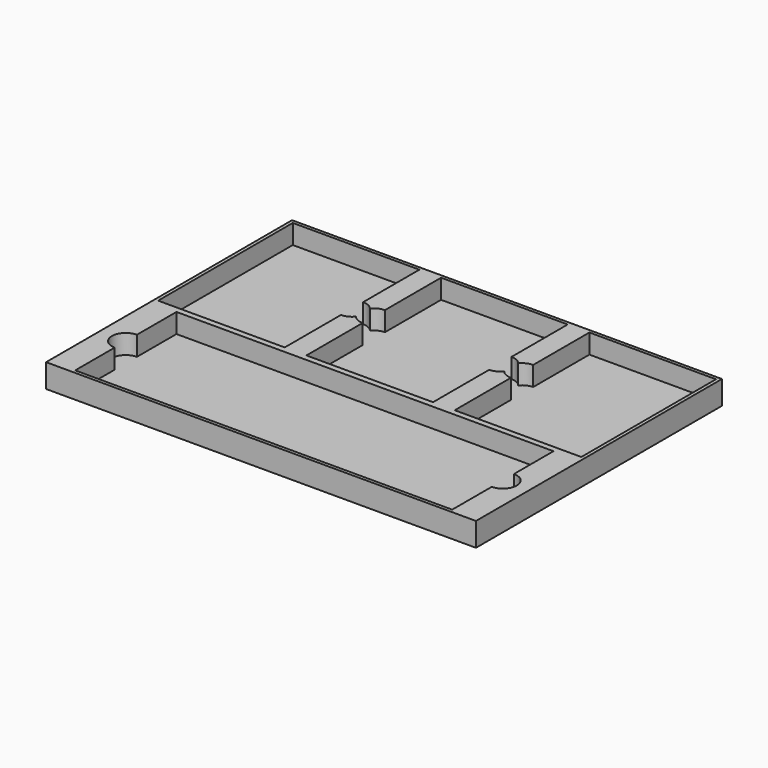
from build123d import *

# Parameters (mm, degrees)
F1_DEPTH = 3
F2_DEPTH = 17


# Not quite as in the source:
# - ends of sketch curves that miss each other by under 0.0002 mm in the source are joined


with BuildPart() as f1:
    # F0 (on Top) → F1 (new body)
    with BuildSketch(Plane.XY):
        Polygon((154.5, 110.5), (-154.5, 110.5), (-154.4999927282, -110.5), (154.5, -110.5), align=None)
        with BuildLine():
            Line((135.5, -108.0998892117), (-135.5, -108.0998892117))
            Line((-135.5, -108.0998892117), (-135.5, -72.5998892117))
            ThreePointArc((-135.5, -72.5998892117), (-145.5, -62.5998892117), (-135.5, -52.5998892117))
            Line((-135.5, -52.5998892117), (-135.5, -17.0998892117))
            Line((-135.5, -17.0998892117), (135.5, -17.0998892117))
            Line((135.5, -17.0998892117), (135.5, -52.5998892117))
            ThreePointArc((135.5, -52.5998892117), (142.5710678119, -55.5288213998), (145.5, -62.5998892117))
            ThreePointArc((145.5, -62.5998892117), (142.5710678119, -69.6709570235), (135.5, -72.5998892117))
            Line((135.5, -72.5998892117), (135.5, -108.0998892117))
        make_face(mode=Mode.SUBTRACT)
        with BuildLine():
            Line((-45.4999990761, 57.6660784096), (-45.4999990761, 108.1660784096))
            Line((-45.4999990761, 108.1660784096), (45.5000009239, 108.1660784096))
            Line((45.5000009239, 108.1660784096), (45.5000009239, 57.6660784096))
            ThreePointArc((45.5000009239, 57.6660784096), (49.8255857676, 56.6821371804), (53.2999463577, 53.9239415616))
            ThreePointArc((53.2999463577, 53.9239415616), (56.7743069478, 56.6821371804), (61.0998917915, 57.6660784096))
            Line((61.0998917915, 57.6660784096), (61.0998917915, 108.1660784096))
            Line((61.0998917915, 108.1660784096), (152.0998917915, 108.1660784096))
            Line((152.0998917915, 108.1660784096), (152.0998917915, -12.8339215904))
            Line((152.0998917915, -12.8339215904), (61.0998917915, -12.8339215904))
            Line((61.0998917915, -12.8339215904), (61.0998917915, 37.6660784096))
            ThreePointArc((61.0998917915, 37.6660784096), (56.7743069478, 38.6500196387), (53.2999463577, 41.4082152575))
            ThreePointArc((53.2999463577, 41.4082152575), (49.8255857676, 38.6500196387), (45.5000009239, 37.6660784096))
            Line((45.5000009239, 37.6660784096), (45.5000009239, -12.8339215904))
            Line((45.5000009239, -12.8339215904), (-45.4999990761, -12.8339215904))
            Line((-45.4999990761, -12.8339215904), (-45.4999990761, 37.6660784096))
            ThreePointArc((-45.4999990761, 37.6660784096), (-49.8257290565, 38.6500892715), (-53.3001459795, 41.4084663822))
            ThreePointArc((-53.3001459795, 41.4084663822), (-56.7745629026, 38.6500892715), (-61.1002928829, 37.6660784096))
            Line((-61.1002928829, 37.6660784096), (-61.1002928829, -12.8339215904))
            Line((-61.1002928829, -12.8339215904), (-152.1002928829, -12.8339215904))
            Line((-152.1002928829, -12.8339215904), (-152.1002928829, 108.1660784096))
            Line((-152.1002928829, 108.1660784096), (-61.1002928829, 108.1660784096))
            Line((-61.1002928829, 108.1660784096), (-61.1002928829, 57.6660784096))
            ThreePointArc((-61.1002928829, 57.6660784096), (-56.7745629026, 56.6820675476), (-53.3001459795, 53.923690437))
            ThreePointArc((-53.3001459795, 53.923690437), (-49.8257290565, 56.6820675476), (-45.4999990761, 57.6660784096))
        make_face(mode=Mode.SUBTRACT)
        with BuildLine():
            Line((-135.5, -72.5998892117), (-135.5, -108.0998892117))
            Line((-135.5, -108.0998892117), (135.5, -108.0998892117))
            Line((135.5, -108.0998892117), (135.5, -72.5998892117))
            ThreePointArc((135.5, -72.5998892117), (125.5, -62.5998892117), (135.5, -52.5998892117))
            Line((135.5, -52.5998892117), (135.5, -17.0998892117))
            Line((135.5, -17.0998892117), (-135.5, -17.0998892117))
            Line((-135.5, -17.0998892117), (-135.5, -52.5998892117))
            ThreePointArc((-135.5, -52.5998892117), (-128.4289321881, -55.5288213998), (-125.5, -62.5998892117))
            ThreePointArc((-125.5, -62.5998892117), (-128.4289321881, -69.6709570235), (-135.5, -72.5998892117))
        make_face()
        with BuildLine():
            ThreePointArc((-61.1002928829, 37.6660784096), (-71.1002928829, 47.6660784096), (-61.1002928829, 57.6660784096))
            Line((-61.1002928829, 57.6660784096), (-61.1002928829, 108.1660784096))
            Line((-61.1002928829, 108.1660784096), (-152.1002928829, 108.1660784096))
            Line((-152.1002928829, 108.1660784096), (-152.1002928829, -12.8339215904))
            Line((-152.1002928829, -12.8339215904), (-61.1002928829, -12.8339215904))
            Line((-61.1002928829, -12.8339215904), (-61.1002928829, 37.6660784096))
        make_face()
        with BuildLine():
            Line((61.0998917915, 108.1660784096), (61.0998917915, 57.6660784096))
            ThreePointArc((61.0998917915, 57.6660784096), (68.1709596034, 54.7371462214), (71.0998917915, 47.6660784096))
            ThreePointArc((71.0998917915, 47.6660784096), (68.1709596034, 40.5950105977), (61.0998917915, 37.6660784096))
            Line((61.0998917915, 37.6660784096), (61.0998917915, -12.8339215904))
            Line((61.0998917915, -12.8339215904), (152.0998917915, -12.8339215904))
            Line((152.0998917915, -12.8339215904), (152.0998917915, 108.1660784096))
            Line((152.0998917915, 108.1660784096), (61.0998917915, 108.1660784096))
        make_face()
        with BuildLine():
            Line((45.5000009239, 108.1660784096), (-45.4999990761, 108.1660784096))
            Line((-45.4999990761, 108.1660784096), (-45.4999990761, 57.6660784096))
            ThreePointArc((-45.4999990761, 57.6660784096), (-38.4289312643, 54.7371462214), (-35.4999990761, 47.6660784096))
            ThreePointArc((-35.4999990761, 47.6660784096), (-38.4289312643, 40.5950105977), (-45.4999990761, 37.6660784096))
            Line((-45.4999990761, 37.6660784096), (-45.4999990761, -12.8339215904))
            Line((-45.4999990761, -12.8339215904), (45.5000009239, -12.8339215904))
            Line((45.5000009239, -12.8339215904), (45.5000009239, 37.6660784096))
            ThreePointArc((45.5000009239, 37.6660784096), (35.5000009239, 47.6660784096), (45.5000009239, 57.6660784096))
            Line((45.5000009239, 57.6660784096), (45.5000009239, 108.1660784096))
        make_face()
        with BuildLine():
            Line((-61.1002928829, 37.6660784096), (-61.1002928829, 57.6660784096))
            ThreePointArc((-61.1002928829, 57.6660784096), (-71.1002928829, 47.6660784096), (-61.1002928829, 37.6660784096))
        make_face()
        with BuildLine():
            Line((45.5000009239, 37.6660784096), (45.5000009239, 57.6660784096))
            ThreePointArc((45.5000009239, 57.6660784096), (35.5000009239, 47.6660784096), (45.5000009239, 37.6660784096))
        make_face()
        with BuildLine():
            ThreePointArc((71.0998917915, 47.6660784096), (68.1709596034, 54.7371462214), (61.0998917915, 57.6660784096))
            Line((61.0998917915, 57.6660784096), (61.0998917915, 37.6660784096))
            ThreePointArc((61.0998917915, 37.6660784096), (68.1709596034, 40.5950105977), (71.0998917915, 47.6660784096))
        make_face()
        with BuildLine():
            Line((135.5, -52.5998892117), (135.5, -72.5998892117))
            ThreePointArc((135.5, -72.5998892117), (142.5710678119, -69.6709570235), (145.5, -62.5998892117))
            ThreePointArc((145.5, -62.5998892117), (142.5710678119, -55.5288213998), (135.5, -52.5998892117))
        make_face()
        with BuildLine():
            ThreePointArc((-35.4999990761, 47.6660784096), (-38.4289312643, 54.7371462214), (-45.4999990761, 57.6660784096))
            Line((-45.4999990761, 57.6660784096), (-45.4999990761, 37.6660784096))
            ThreePointArc((-45.4999990761, 37.6660784096), (-38.4289312643, 40.5950105977), (-35.4999990761, 47.6660784096))
        make_face()
        with BuildLine():
            ThreePointArc((135.5, -52.5998892117), (125.5, -62.5998892117), (135.5, -72.5998892117))
            Line((135.5, -72.5998892117), (135.5, -52.5998892117))
        make_face()
        with BuildLine():
            Line((-135.5, -52.5998892117), (-135.5, -72.5998892117))
            ThreePointArc((-135.5, -72.5998892117), (-128.4289321881, -69.6709570235), (-125.5, -62.5998892117))
            ThreePointArc((-125.5, -62.5998892117), (-128.4289321881, -55.5288213998), (-135.5, -52.5998892117))
        make_face()
        with BuildLine():
            ThreePointArc((-135.5, -52.5998892117), (-145.5, -62.5998892117), (-135.5, -72.5998892117))
            Line((-135.5, -72.5998892117), (-135.5, -52.5998892117))
        make_face()
        with BuildLine():
            Line((-45.4999990761, 37.6660784096), (-45.4999990761, 57.6660784096))
            ThreePointArc((-45.4999990761, 57.6660784096), (-49.8257290565, 56.6820675476), (-53.3001459795, 53.923690437))
            ThreePointArc((-53.3001459795, 53.923690437), (-51.6662728216, 50.9825924655), (-51.1002928829, 47.6660784096))
            ThreePointArc((-51.1002928829, 47.6660784096), (-51.6662728216, 44.3495643536), (-53.3001459795, 41.4084663822))
            ThreePointArc((-53.3001459795, 41.4084663822), (-49.8257290565, 38.6500892715), (-45.4999990761, 37.6660784096))
        make_face()
        with BuildLine():
            ThreePointArc((-53.3001459795, 41.4084663822), (-55.4999990761, 47.6660784096), (-53.3001459795, 53.923690437))
            ThreePointArc((-53.3001459795, 53.923690437), (-56.7745629026, 56.6820675476), (-61.1002928829, 57.6660784096))
            Line((-61.1002928829, 57.6660784096), (-61.1002928829, 37.6660784096))
            ThreePointArc((-61.1002928829, 37.6660784096), (-56.7745629026, 38.6500892715), (-53.3001459795, 41.4084663822))
        make_face()
        with BuildLine():
            ThreePointArc((61.0998917915, 57.6660784096), (56.7743069478, 56.6821371804), (53.2999463577, 53.9239415616))
            ThreePointArc((53.2999463577, 53.9239415616), (54.9339675959, 50.9827443305), (55.5000009239, 47.6660784096))
            ThreePointArc((55.5000009239, 47.6660784096), (54.9339675959, 44.3494124887), (53.2999463577, 41.4082152575))
            ThreePointArc((53.2999463577, 41.4082152575), (56.7743069478, 38.6500196387), (61.0998917915, 37.6660784096))
            Line((61.0998917915, 37.6660784096), (61.0998917915, 57.6660784096))
        make_face()
        with BuildLine():
            ThreePointArc((53.2999463577, 53.9239415616), (49.8255857676, 56.6821371804), (45.5000009239, 57.6660784096))
            Line((45.5000009239, 57.6660784096), (45.5000009239, 37.6660784096))
            ThreePointArc((45.5000009239, 37.6660784096), (49.8255857676, 38.6500196387), (53.2999463577, 41.4082152575))
            ThreePointArc((53.2999463577, 41.4082152575), (51.0998917915, 47.6660784096), (53.2999463577, 53.9239415616))
        make_face()
        with BuildLine():
            ThreePointArc((55.5000009239, 47.6660784096), (54.9339675959, 50.9827443305), (53.2999463577, 53.9239415616))
            ThreePointArc((53.2999463577, 53.9239415616), (51.0998917915, 47.6660784096), (53.2999463577, 41.4082152575))
            ThreePointArc((53.2999463577, 41.4082152575), (54.9339675959, 44.3494124887), (55.5000009239, 47.6660784096))
        make_face()
        with BuildLine():
            ThreePointArc((-51.1002928829, 47.6660784096), (-51.6662728216, 50.9825924655), (-53.3001459795, 53.923690437))
            ThreePointArc((-53.3001459795, 53.923690437), (-55.4999990761, 47.6660784096), (-53.3001459795, 41.4084663822))
            ThreePointArc((-53.3001459795, 41.4084663822), (-51.6662728216, 44.3495643536), (-51.1002928829, 47.6660784096))
        make_face()
    extrude(amount=F1_DEPTH)

    # F0 (on Top) → F2 (join)
    with BuildSketch(Plane.XY):
        Polygon((154.5, 110.5), (-154.5, 110.5), (-154.4999927282, -110.5), (154.5, -110.5), align=None)
        with BuildLine():
            Line((135.5, -108.0998892117), (-135.5, -108.0998892117))
            Line((-135.5, -108.0998892117), (-135.5, -72.5998892117))
            ThreePointArc((-135.5, -72.5998892117), (-145.5, -62.5998892117), (-135.5, -52.5998892117))
            Line((-135.5, -52.5998892117), (-135.5, -17.0998892117))
            Line((-135.5, -17.0998892117), (135.5, -17.0998892117))
            Line((135.5, -17.0998892117), (135.5, -52.5998892117))
            ThreePointArc((135.5, -52.5998892117), (142.5710678119, -55.5288213998), (145.5, -62.5998892117))
            ThreePointArc((145.5, -62.5998892117), (142.5710678119, -69.6709570235), (135.5, -72.5998892117))
            Line((135.5, -72.5998892117), (135.5, -108.0998892117))
        make_face(mode=Mode.SUBTRACT)
        with BuildLine():
            Line((-45.4999990761, 57.6660784096), (-45.4999990761, 108.1660784096))
            Line((-45.4999990761, 108.1660784096), (45.5000009239, 108.1660784096))
            Line((45.5000009239, 108.1660784096), (45.5000009239, 57.6660784096))
            ThreePointArc((45.5000009239, 57.6660784096), (49.8255857676, 56.6821371804), (53.2999463577, 53.9239415616))
            ThreePointArc((53.2999463577, 53.9239415616), (56.7743069478, 56.6821371804), (61.0998917915, 57.6660784096))
            Line((61.0998917915, 57.6660784096), (61.0998917915, 108.1660784096))
            Line((61.0998917915, 108.1660784096), (152.0998917915, 108.1660784096))
            Line((152.0998917915, 108.1660784096), (152.0998917915, -12.8339215904))
            Line((152.0998917915, -12.8339215904), (61.0998917915, -12.8339215904))
            Line((61.0998917915, -12.8339215904), (61.0998917915, 37.6660784096))
            ThreePointArc((61.0998917915, 37.6660784096), (56.7743069478, 38.6500196387), (53.2999463577, 41.4082152575))
            ThreePointArc((53.2999463577, 41.4082152575), (49.8255857676, 38.6500196387), (45.5000009239, 37.6660784096))
            Line((45.5000009239, 37.6660784096), (45.5000009239, -12.8339215904))
            Line((45.5000009239, -12.8339215904), (-45.4999990761, -12.8339215904))
            Line((-45.4999990761, -12.8339215904), (-45.4999990761, 37.6660784096))
            ThreePointArc((-45.4999990761, 37.6660784096), (-49.8257290565, 38.6500892715), (-53.3001459795, 41.4084663822))
            ThreePointArc((-53.3001459795, 41.4084663822), (-56.7745629026, 38.6500892715), (-61.1002928829, 37.6660784096))
            Line((-61.1002928829, 37.6660784096), (-61.1002928829, -12.8339215904))
            Line((-61.1002928829, -12.8339215904), (-152.1002928829, -12.8339215904))
            Line((-152.1002928829, -12.8339215904), (-152.1002928829, 108.1660784096))
            Line((-152.1002928829, 108.1660784096), (-61.1002928829, 108.1660784096))
            Line((-61.1002928829, 108.1660784096), (-61.1002928829, 57.6660784096))
            ThreePointArc((-61.1002928829, 57.6660784096), (-56.7745629026, 56.6820675476), (-53.3001459795, 53.923690437))
            ThreePointArc((-53.3001459795, 53.923690437), (-49.8257290565, 56.6820675476), (-45.4999990761, 57.6660784096))
        make_face(mode=Mode.SUBTRACT)
    extrude(amount=F2_DEPTH)


solid = f1.part
